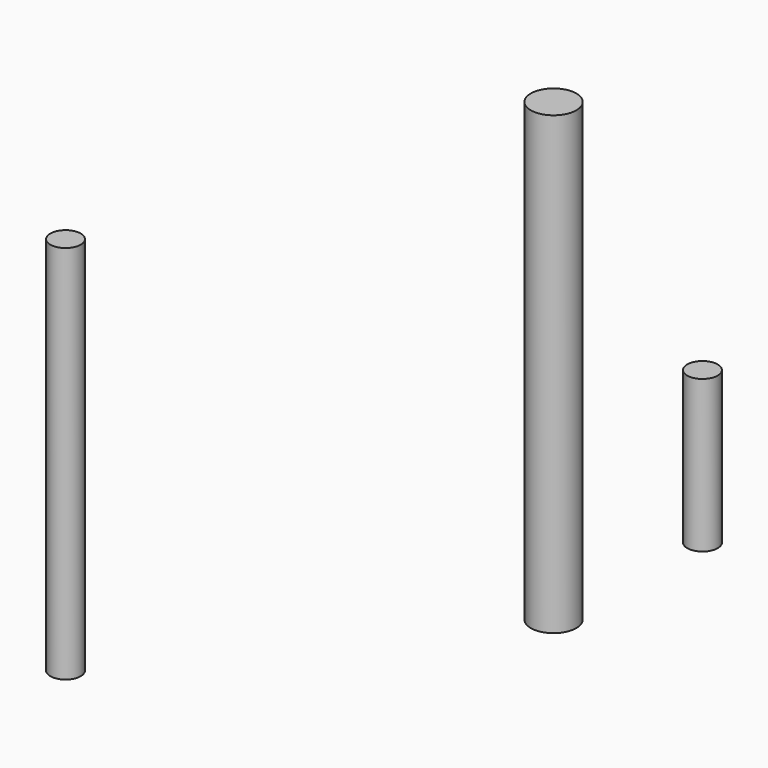
from build123d import *

# Parameters (mm, degrees)
F0_R     = 1
F1_DEPTH = 25
F2_R     = 1
F3_DEPTH = 10
F4_R     = 1.5
F5_DEPTH = 30


# Not quite as in the source:
# - a feature names something its author has since deleted; it is built from what else it names


with BuildPart() as f1:
    # F0 (on Top) → F1 (new body)
    with BuildSketch(Plane.XY):
        with Locations((26.4221140966, 32.5091108651)):
            Circle(F0_R)
    extrude(amount=F1_DEPTH)


with BuildPart() as f3:
    # F2 (on Top) → F3 (new body)
    with BuildSketch(Plane.XY):
        with Locations((43.0808849633, 64.0808865428)):
            Circle(F2_R)
    extrude(amount=F3_DEPTH)


with BuildPart() as f5:
    # F4 (on Top) → F5 (new body)
    with BuildSketch(Plane.XY):
        with Locations((42.4658991396, 52.6014268398)):
            Circle(F4_R)
    extrude(amount=F5_DEPTH)


solid = Compound([f1.part, f3.part, f5.part])
